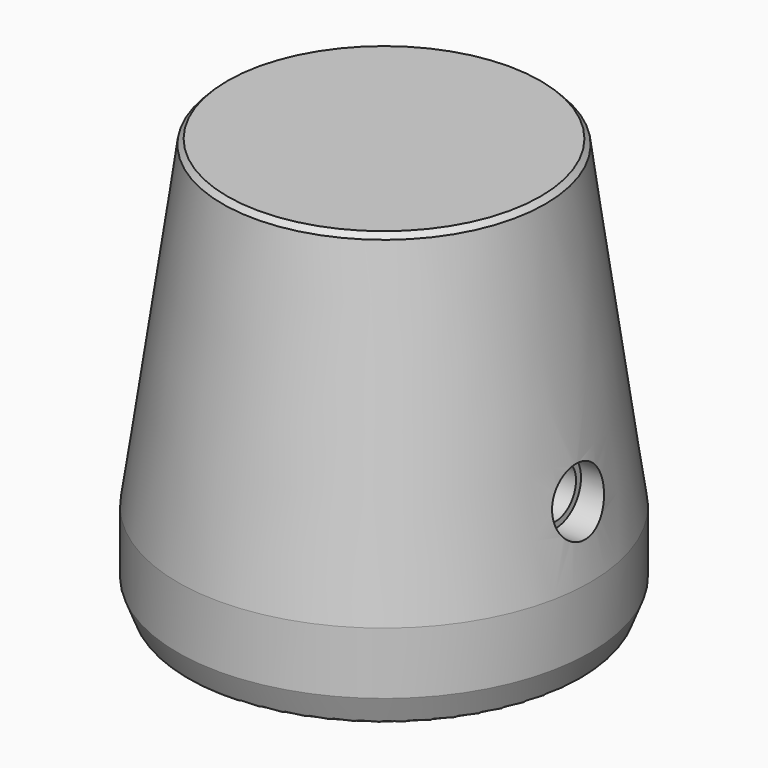
from build123d import *

# Parameters (mm, degrees)
F3_SIZE        = 1
F4_SIZE2       = 0.2
F4_SIZE        = 0.25
F5_R           = 0.1524
F8_D           = 2.5
F8_DEPTH       = 10
F8_START       = 0.6846642
F8_CBORE_D     = 3.1
F8_CBORE_DEPTH = 1
F8_TIP         = 0.7510757738
F9_R           = 2.78
F10_DEPTH      = 2.15


with BuildPart() as f2:
    # F1 (on Front) → F2 (revolve)
    with BuildSketch(Plane.XZ):
        Polygon((6.8, 4.2), (6.8, 0), (9.5, 0), (10, 1.3), (10, 4.3), (7.7935088952, 20), (0, 20), (0, 18), (1.61, 18), (1.61, 4.2), align=None)
    revolve(axis=Axis((0, 0, 12.1), (0, 0, 1)))

    # F3
    f3_edges = [f2.edges().sort_by_distance(p)[0] for p in [
        (-1.61, 0, 18),
    ]]
    chamfer(f3_edges, length=F3_SIZE)

    # F4
    f4_edges = [f2.edges().sort_by_distance(p)[0] for p in [
        (-7.793509, 0, 20),
    ]]
    chamfer(f4_edges, length=F4_SIZE, length2=F4_SIZE2)

    # F5
    f5_edges = [f2.edges().sort_by_distance(p)[0] for p in [
        (-6.8, 0, 0),
        (-9.5, 0, 0),
        (-6.8, 0, 4.2),
        (-1.61, 0, 4.2),
    ]]
    fillet(f5_edges, radius=F5_R)

    # F8
    # its depths count from where the whole tool has entered the part; down to there all is cleared
    with Locations(Plane.YZ.offset(10).offset(-F8_START)):
        with Locations((0, 7.6)):
            CounterBoreHole(F8_D / 2, F8_CBORE_D / 2, F8_CBORE_DEPTH, depth=F8_DEPTH)
            with Locations((0, 0, -(F8_DEPTH + F8_TIP / 2))):  # 118° drill point
                Cone(0, F8_D / 2, F8_TIP, mode=Mode.SUBTRACT)


with BuildPart() as f10:
    # F9 (on Top) → F10 (new body)
    with BuildSketch(Plane.XY):
        Polygon((-2.3036275741, -3.99), (2.3036275741, -3.99), (4.6072551481, 0), (2.3036275741, 3.99), (-2.3036275741, 3.99), (-4.6072551481, 0), align=None)
        Circle(F9_R, mode=Mode.SUBTRACT)
    extrude(amount=F10_DEPTH)


solid = Compound([f2.part, f10.part])
